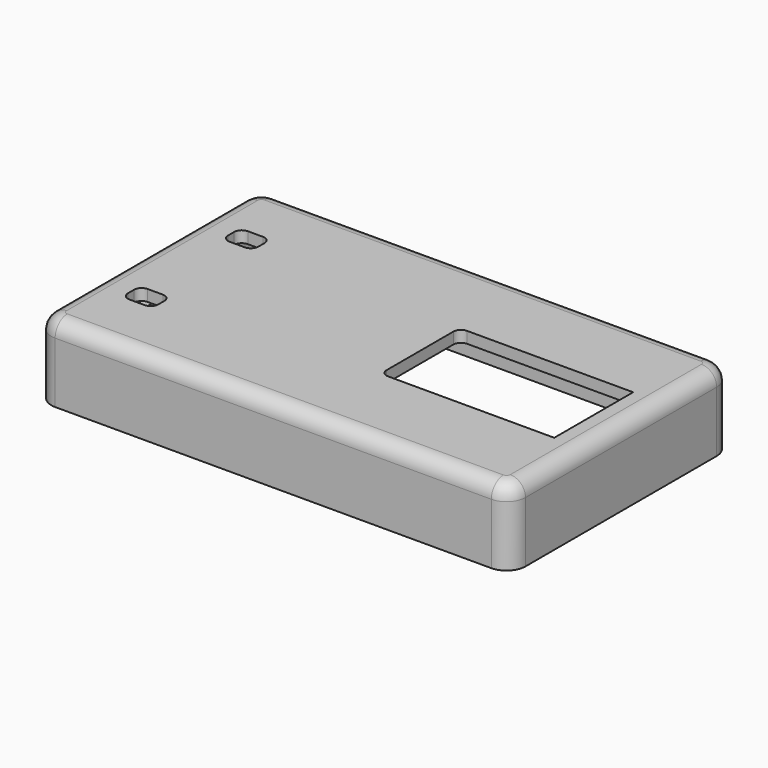
from build123d import *

# Parameters (mm, degrees)
F0_W          = 62.5
F0_H          = 36.5
F0_W_2        = 58.5
F0_H_2        = 31.5
F1_DEPTH      = 7
F2_W          = 4
F2_H          = 3
F2_W_2        = 2.1059160829
F2_H_2        = 13
F3_DEPTH      = 1.5
F4_W          = 62.5
F4_H          = 36.5
F5_DEPTH      = 3
F7_DEPTH      = 2.5
F8_R          = 2.5
F9_R          = 1
F11_T1_DEPTH  = 57.5
F11_T3_DEPTH  = 31.5
F11_T6_ANGLE  = 90
F11_T8_ANGLE  = 90
F11_T10_ANGLE = 90
F11_T12_ANGLE = 90
F12_W         = 1.25
F12_H         = 8.5
F13_DEPTH     = 2


# Not quite as in the source:
# - a fillet or chamfer that OpenCascade refuses, or shapes differently, is made with other operations: its cross-section is extruded or revolved along the edge and cut away or added
# - two fillets or chamfers of one size are made in one step


with BuildPart() as f1:
    # F0 (on Top) → F1 (new body)
    with BuildSketch(Plane.XY):
        with Locations((0.5, 0.5)):
            Rectangle(F0_W, F0_H)
        with Locations((1, 0.5)):
            Rectangle(F0_W_2, F0_H_2, mode=Mode.SUBTRACT)
    extrude(amount=F1_DEPTH)

    # F2 (on face) → F3 (join)
    with BuildSketch(Plane.XY.offset(7)):
        Polygon((30.25, 16.25), (-28.25, 16.25), (-28.25, -15.25), (30.25, -15.25), (30.25, -6), (28.1440839171, -6), (5.25, -6), (5.25, 7), (28.1440839171, 7), (30.25, 7), align=None)
        with Locations((-24.25, -7.75)):
            Rectangle(F2_W, F2_H, mode=Mode.SUBTRACT)
        with Locations((-24.25, 8.75)):
            Rectangle(F2_W, F2_H, mode=Mode.SUBTRACT)
        with Locations((29.1970419586, 0.5)):
            Rectangle(F2_W_2, F2_H_2)
    extrude(amount=-F3_DEPTH)

    # F4 (on face) → F5 (join)
    with BuildSketch(Plane(origin=(0, 0, 0), x_dir=(1, 0, 0), z_dir=(0, 0, -1))):
        with Locations((0.5, -0.5)):
            Rectangle(F4_W, F4_H)
        Polygon((-29.5, -17.522141248), (-29.5, 16.5), (30.25, 16.5), (30.25, 15.25), (30.25, -16.25), (30.25, -17.522141248), align=None, mode=Mode.SUBTRACT)
    extrude(amount=F5_DEPTH)

    # F6 (on face) → F7 (cut)
    with BuildSketch(Plane.YZ.offset(-28.25)):
        with BuildLine():
            Line((4, 5.5), (-3, 5.5))
            ThreePointArc((-3, 5.5), (-3.5303300859, 5.2803300859), (-3.75, 4.75))
            Line((-3.75, 4.75), (-3.75, 3.5))
            ThreePointArc((-3.75, 3.5), (-3.1642135624, 2.0857864376), (-1.75, 1.5))
            Line((-1.75, 1.5), (2.75, 1.5))
            ThreePointArc((2.75, 1.5), (4.1642135624, 2.0857864376), (4.75, 3.5))
            Line((4.75, 3.5), (4.75, 4.75))
            ThreePointArc((4.75, 4.75), (4.5303300859, 5.2803300859), (4, 5.5))
        make_face()
    extrude(amount=-F7_DEPTH, mode=Mode.SUBTRACT)

    # F8
    f8_edges = [f1.edges().sort_by_distance(p)[0] for p in [
        (-30.75, 18.75, 2),
        (-30.75, -17.75, 2),
        (31.75, 18.75, 2),
        (31.75, -17.75, 2),
    ]]
    fillet(f8_edges, radius=F8_R)

    # F9
    f9_edges = [f1.edges().sort_by_distance(p)[0] for p in [
        (5.25, 7, 6.25),
        (5.25, -6, 6.25),
        (-22.25, 10.25, 6.25),
        (-22.25, 7.25, 6.25),
        (-26.25, 7.25, 6.25),
        (-26.25, 10.25, 6.25),
        (-26.25, -9.25, 6.25),
        (-26.25, -6.25, 6.25),
        (-22.25, -6.25, 6.25),
        (-22.25, -9.25, 6.25),
    ]]
    fillet(f9_edges, radius=F9_R)

    # F11: fillet of radius 2 on 8 edges, made by hand

    # F11_s2 → F11_t1 (cut)
    with BuildSketch(Plane.YZ.offset(-28.25)):
        with BuildLine():
            ThreePointArc((-15.75, 7), (-17.1642135624, 6.4142135624), (-17.75, 5))
            Line((-17.75, 5), (-17.75, 7))
            Line((-17.75, 7), (-15.75, 7))
        make_face()
        with BuildLine():
            ThreePointArc((16.75, 7), (18.1642135624, 6.4142135624), (18.75, 5))
            Line((18.75, 5), (18.75, 7))
            Line((18.75, 7), (16.75, 7))
        make_face()
    extrude(amount=F11_T1_DEPTH, mode=Mode.SUBTRACT)

    # F11_s4 → F11_t3 (cut)
    with BuildSketch(Plane.XZ.offset(-16.25)):
        with BuildLine():
            ThreePointArc((29.75, 7), (31.1642135624, 6.4142135624), (31.75, 5))
            Line((31.75, 5), (31.75, 7))
            Line((31.75, 7), (29.75, 7))
        make_face()
        with BuildLine():
            ThreePointArc((-28.75, 7), (-30.1642135624, 6.4142135624), (-30.75, 5))
            Line((-30.75, 5), (-30.75, 7))
            Line((-30.75, 7), (-28.75, 7))
        make_face()
    extrude(amount=F11_T3_DEPTH, mode=Mode.SUBTRACT)

    # F11_s5 → F11_t6 (revolve, cut)
    with BuildSketch(Plane.YZ.offset(29.25)):
        with BuildLine():
            ThreePointArc((16.75, 7), (18.1642135624, 6.4142135624), (18.75, 5))
            Line((18.75, 5), (18.75, 7))
            Line((18.75, 7), (16.75, 7))
        make_face()
    revolve(axis=Axis((29.25, 16.25, 7), (0, 0, -1)), revolution_arc=F11_T6_ANGLE, mode=Mode.SUBTRACT)

    # F11_s7 → F11_t8 (revolve, cut)
    with BuildSketch(Plane.YZ.offset(-28.25)):
        with BuildLine():
            ThreePointArc((16.75, 7), (18.1642135624, 6.4142135624), (18.75, 5))
            Line((18.75, 5), (18.75, 7))
            Line((18.75, 7), (16.75, 7))
        make_face()
    revolve(axis=Axis((-28.25, 16.25, 7), (0, 0, 1)), revolution_arc=F11_T8_ANGLE, mode=Mode.SUBTRACT)

    # F11_s9 → F11_t10 (revolve, cut)
    with BuildSketch(Plane.XZ.offset(15.25)):
        with BuildLine():
            ThreePointArc((29.75, 7), (31.1642135624, 6.4142135624), (31.75, 5))
            Line((31.75, 5), (31.75, 7))
            Line((31.75, 7), (29.75, 7))
        make_face()
    revolve(axis=Axis((29.25, -15.25, 7), (0, 0, -1)), revolution_arc=F11_T10_ANGLE, mode=Mode.SUBTRACT)

    # F11_s11 → F11_t12 (revolve, cut)
    with BuildSketch(Plane.XZ.offset(15.25)):
        with BuildLine():
            ThreePointArc((-28.75, 7), (-30.1642135624, 6.4142135624), (-30.75, 5))
            Line((-30.75, 5), (-30.75, 7))
            Line((-30.75, 7), (-28.75, 7))
        make_face()
    revolve(axis=Axis((-28.25, -15.25, 7), (0, 0, 1)), revolution_arc=F11_T12_ANGLE, mode=Mode.SUBTRACT)

    # F12 (on face) → F13 (cut)
    with BuildSketch(Plane(origin=(0, 0, 0), x_dir=(1, 0, 0), z_dir=(0, 0, -1))):
        with Locations((-28.875, -0.5)):
            Rectangle(F12_W, F12_H)
    extrude(amount=-F13_DEPTH, mode=Mode.SUBTRACT)


solid = f1.part
